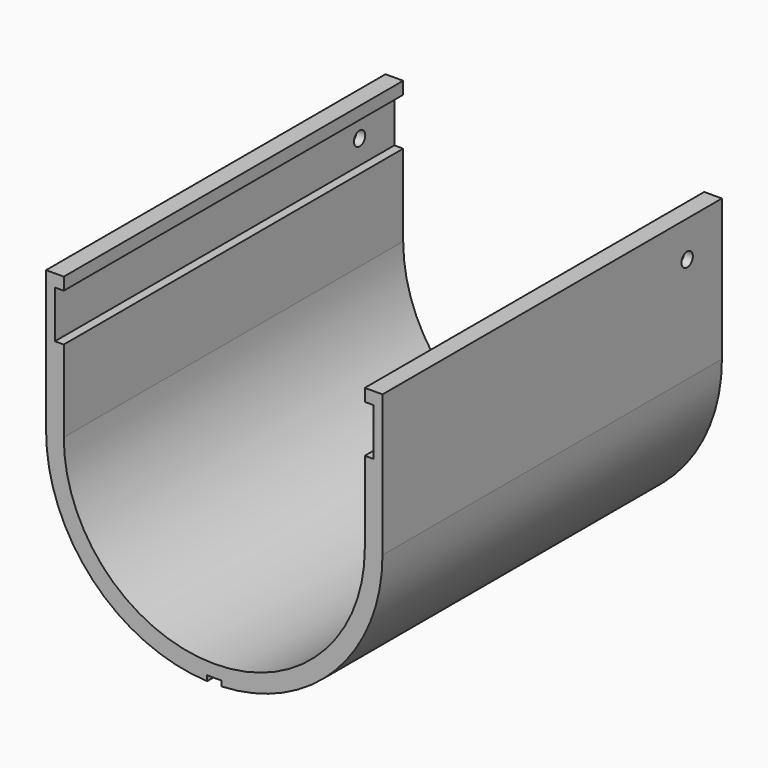
from build123d import *

# Parameters (mm, degrees)
F1_DEPTH = 120
F2_R     = 2
F3_DEPTH = 95.141


# Not quite as in the source:
# - ends of sketch curves that miss each other by under 0.0002 mm in the source are joined


with BuildPart() as f1:
    # F0 (on Front) → F1 (new body)
    with BuildSketch(Plane.XZ):
        with BuildLine():
            Line((-42.5699986517, 0), (-47.569999482, 0))
            Line((-47.569999482, 0), (-47.569999482, -40))
            ThreePointArc((-47.569999482, -40), (-34.336896153, -72.9223698712), (-2, -87.5279378404))
            Line((-2, -87.5279378404), (-2, -86.0265670688))
            ThreePointArc((-2, -86.0265670688), (0, -86.069999741), (2, -86.0265670688))
            Line((2, -86.0265670688), (2, -87.5279378404))
            ThreePointArc((2, -87.5279378404), (34.336896153, -72.9223698712), (47.569999741, -40))
            Line((47.569999741, -40), (47.570000518, 0))
            Line((47.570000518, 0), (42.570000518, 0))
            Line((42.570000518, 0), (42.570000518, -3.5))
            Line((42.570000518, -3.5), (45.070000518, -3.5))
            Line((45.070000518, -3.5), (45.070000518, -16.9))
            Line((45.070000518, -16.9), (42.570000518, -16.9))
            Line((42.570000518, -16.9), (42.570000518, -40))
            ThreePointArc((42.570000518, -40), (0, -82.5699996948), (-42.5699996948, -40))
            Line((-42.5699996948, -40), (-42.5699986517, -16.9))
            Line((-42.5699986517, -16.9), (-45.070000518, -16.9))
            Line((-45.070000518, -16.9), (-45.070000518, -3.5))
            Line((-45.070000518, -3.5), (-42.5699986517, -3.5))
            Line((-42.5699986517, -3.5), (-42.5699986517, 0))
        make_face()
    extrude(amount=F1_DEPTH)

    # F2 (on face) → F3 (cut, through all)
    with BuildSketch(Plane.YZ.offset(47.570000518)):
        with Locations((-12.29, -10.2)):
            Circle(F2_R)
    extrude(amount=-F3_DEPTH, mode=Mode.SUBTRACT)


solid = f1.part
